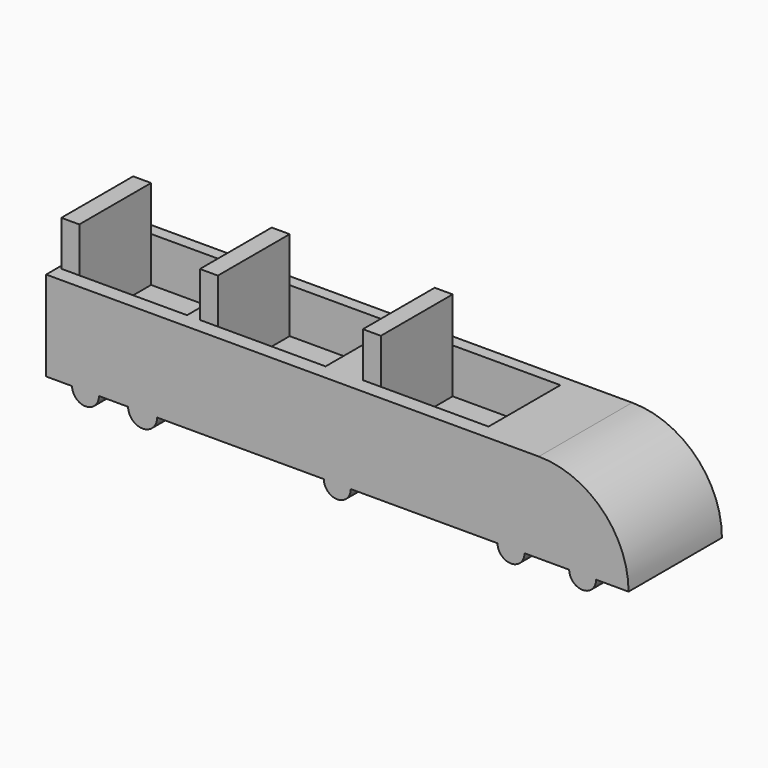
from build123d import *

# Parameters (mm, degrees)
F0_W      = 324.4502871967
F0_H      = 65
F1_DEPTH  = 50
F2_R      = 49.99999
F3_W      = 60
F3_H      = 50
F4_DEPTH  = 25
F6_DEPTH  = 65
F8_DEPTH  = 65
F9_W      = 10
F9_H      = 50
F10_DEPTH = 25


# Not quite as in the source:
# - a fillet or chamfer is up to 0.001 mm smaller than in the source, because OpenCascade refuses the exact size


with BuildPart() as f1:
    # F0 (on Top) → F1 (new body)
    with BuildSketch(Plane.XY):
        with Locations((69.7921998799, -49.3180742487)):
            Rectangle(F0_W, F0_H)
    extrude(amount=F1_DEPTH)

    # F2 (radius 50 in the source; OpenCascade refuses exactly that, so slightly less here)
    f2_edges = [f1.edges().sort_by_distance(p)[0] for p in [
        (232.017343, -49.318074, 50),
    ]]
    fillet(f2_edges, radius=F2_R)

    # F3 (on face) → F4 (cut)
    with BuildSketch(Plane.XY.offset(50)):
        with Locations((-50.6331702159, -48.4395725653)):
            Rectangle(F3_W, F3_H)
        with Locations((26.5513133067, -48.4395725653)):
            Rectangle(F3_W, F3_H)
        with Locations((117.3280163615, -48.4395725653)):
            Rectangle(F3_W, F3_H)
    extrude(amount=-F4_DEPTH, mode=Mode.SUBTRACT)

    # F5 (on face) → F6 (cut)
    with BuildSketch(Plane.XZ.offset(81.8180742487)):
        with BuildLine():
            ThreePointArc((211.8422013521, 0), (204.3422013521, 7.5), (196.8422013521, 0))
            Line((196.8422013521, 0), (211.8422013521, 0))
        make_face()
        with BuildLine():
            ThreePointArc((165.3422039747, 0), (157.8422039747, 7.5), (150.3422039747, 0))
            Line((150.3422039747, 0), (165.3422039747, 0))
        make_face()
        with BuildLine():
            ThreePointArc((-22.1578053385, 0), (-29.6578053385, 7.5), (-37.1578053385, 0))
            Line((-37.1578053385, 0), (-22.1578053385, 0))
        make_face()
        with BuildLine():
            Line((-85.1578038931, 0), (-70.1578038931, 0))
            ThreePointArc((-70.1578038931, 0), (-77.6578038931, 7.5), (-85.1578038931, 0))
        make_face()
    extrude(amount=F6_DEPTH, mode=Mode.SUBTRACT)

    # F7 (on face) → F8 (join)
    with BuildSketch(Plane(origin=(0, -16.8180742487, 0), x_dir=(-1, 0, 0), z_dir=(0, 1, 0))):
        with BuildLine():
            Line((-213.942207098, 0), (-198.942207098, 0))
            ThreePointArc((-198.942207098, 0), (-206.442207098, 7.5), (-213.942207098, 0))
        make_face()
        with BuildLine():
            ThreePointArc((-213.942207098, 0), (-206.442207098, -7.5), (-198.942207098, 0))
            Line((-198.942207098, 0), (-213.942207098, 0))
        make_face()
        with BuildLine():
            Line((-159.0422022343, 0), (-174.0422022343, 0))
            ThreePointArc((-174.0422022343, 0), (-166.5422022343, -7.5), (-159.0422022343, 0))
        make_face()
        with BuildLine():
            ThreePointArc((-159.0422022343, 0), (-166.5422022343, 7.5), (-174.0422022343, 0))
            Line((-174.0422022343, 0), (-159.0422022343, 0))
        make_face()
        with BuildLine():
            Line((-62.2921998799, 0), (-77.2921998799, 0))
            ThreePointArc((-77.2921998799, 0), (-69.7921998799, -7.5), (-62.2921998799, 0))
        make_face()
        with BuildLine():
            ThreePointArc((-62.2921998799, 0), (-69.7921998799, 7.5), (-77.2921998799, 0))
            Line((-77.2921998799, 0), (-62.2921998799, 0))
        make_face()
        with BuildLine():
            Line((46.7355581226, 0), (30.5800629554, 0))
            ThreePointArc((30.5800629554, 0), (38.657810539, -8.0777475836), (46.7355581226, 0))
        make_face()
        with BuildLine():
            ThreePointArc((62.9578086734, 0), (70.4578086734, -7.5), (77.9578086734, 0))
            Line((77.9578086734, 0), (62.9578086734, 0))
        make_face()
    extrude(amount=-F8_DEPTH)

    # F9 (on face) → F10 (join)
    with BuildSketch(Plane.XY.offset(50)):
        with Locations((-85.6331702159, -48.4395725653)):
            Rectangle(F9_W, F9_H)
        with Locations((-8.4486866933, -48.4395725653)):
            Rectangle(F9_W, F9_H)
        with Locations((82.3280163615, -48.4395725653)):
            Rectangle(F9_W, F9_H)
    extrude(amount=F10_DEPTH)


solid = f1.part
